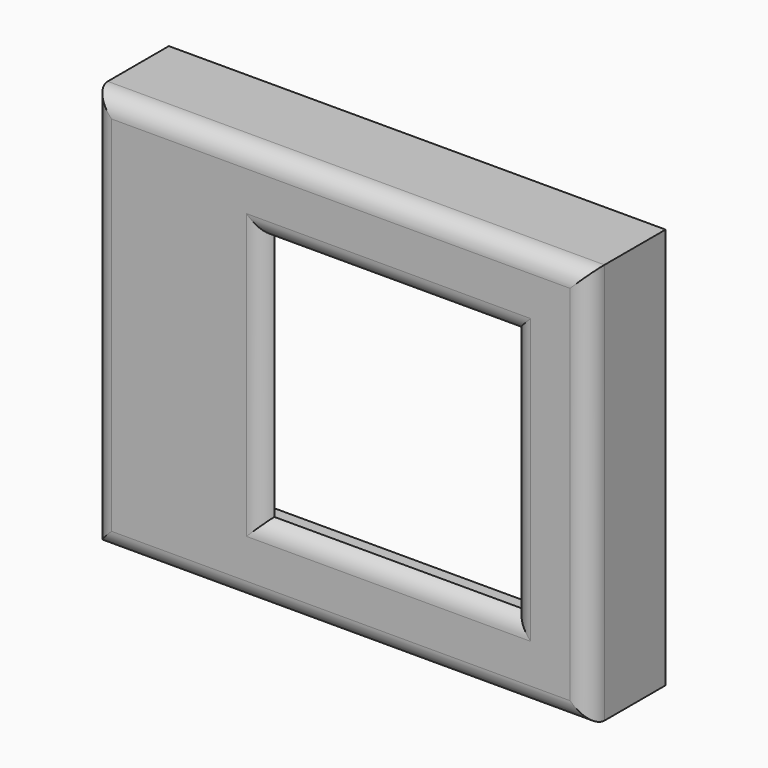
from build123d import *

# Parameters (mm, degrees)
F0_W         = 52
F0_H         = 42
F1_DEPTH     = 10
F2_W         = 26
F2_H         = 26
F3_DEPTH     = 25
F4_W         = 43
F4_H         = 36
F4_W_2       = 26
F4_H_2       = 26
F5_DEPTH     = 8.7
F6_T1_DEPTH  = 52
F6_T3_DEPTH  = 62
F6_T5_DEPTH  = 26
F6_T7_DEPTH  = 26
F6_T13_DEPTH = 30.6837484988
F6_T17_DEPTH = 30.6837484988
F6_T24_DEPTH = 30.6837484988
F6_T28_DEPTH = 30.6837484988
F6_T35_DEPTH = 30.6837484988
F6_T39_DEPTH = 30.6837484988
F6_T46_DEPTH = 30.6837484988
F6_T50_DEPTH = 30.6837484988


# Not quite as in the source:
# - a fillet or chamfer that OpenCascade refuses, or shapes differently, is made with other operations: its cross-section is extruded or revolved along the edge and cut away or added


with BuildPart() as f1:
    # F0 (on Front) → F1 (new body)
    with BuildSketch(Plane.XZ):
        Rectangle(F0_W, F0_H)
    extrude(amount=-F1_DEPTH)

    # F2 (on face) → F3 (cut)
    with BuildSketch(Plane.XZ):
        with Locations((5, 0)):
            Rectangle(F2_W, F2_H)
    extrude(amount=-F3_DEPTH, mode=Mode.SUBTRACT)

    # F4 (on face) → F5 (cut)
    with BuildSketch(Plane(origin=(0, 10, 0), x_dir=(-1, 0, 0), z_dir=(0, 1, 0))):
        with Locations((-1.5, 0)):
            Rectangle(F4_W, F4_H)
        with Locations((-5, 0)):
            Rectangle(F4_W_2, F4_H_2, mode=Mode.SUBTRACT)
    extrude(amount=-F5_DEPTH, mode=Mode.SUBTRACT)

    # F6: fillet of radius 2 on 8 edges, made by hand

    # F6_s2 → F6_t1 (cut)
    with BuildSketch(Plane.XY.offset(-26)):
        with BuildLine():
            ThreePointArc((-26, 2), (-25.4142135624, 0.5857864376), (-24, 0))
            Line((-24, 0), (-26, 0))
            Line((-26, 0), (-26, 2))
        make_face()
        with BuildLine():
            ThreePointArc((26, 2), (25.4142135624, 0.5857864376), (24, 0))
            Line((24, 0), (26, 0))
            Line((26, 0), (26, 2))
        make_face()
    extrude(amount=F6_T1_DEPTH, mode=Mode.SUBTRACT)

    # F6_s4 → F6_t3 (cut)
    with BuildSketch(Plane.YZ.offset(-31)):
        with BuildLine():
            ThreePointArc((0, 19), (0.5857864376, 20.4142135624), (2, 21))
            Line((2, 21), (0, 21))
            Line((0, 21), (0, 19))
        make_face()
        with BuildLine():
            ThreePointArc((2, -21), (0.5857864376, -20.4142135624), (0, -19))
            Line((0, -19), (0, -21))
            Line((0, -21), (2, -21))
        make_face()
    extrude(amount=F6_T3_DEPTH, mode=Mode.SUBTRACT)

    # F6_s6 → F6_t5 (cut)
    with BuildSketch(Plane.XY.offset(-13)):
        with BuildLine():
            ThreePointArc((-9.8734993995, 0), (-8.7333239744, 0.3568323275), (-8, 1.3))
            Line((-8, 1.3), (-8, 0))
            Line((-8, 0), (-9.8734993995, 0))
        make_face()
        with BuildLine():
            ThreePointArc((19.8734993995, 0), (18.7333239744, 0.3568323275), (18, 1.3))
            Line((18, 1.3), (18, 0))
            Line((18, 0), (19.8734993995, 0))
        make_face()
    extrude(amount=F6_T5_DEPTH, mode=Mode.SUBTRACT)

    # F6_s8 → F6_t7 (cut)
    with BuildSketch(Plane.YZ.offset(-8)):
        with BuildLine():
            ThreePointArc((0, -14.8734993995), (0.3568323275, -13.7333239744), (1.3, -13))
            Line((1.3, -13), (0, -13))
            Line((0, -13), (0, -14.8734993995))
        make_face()
        with BuildLine():
            ThreePointArc((0, 14.8734993995), (0.3568323275, 13.7333239744), (1.3, 13))
            Line((1.3, 13), (0, 13))
            Line((0, 13), (0, 14.8734993995))
        make_face()
    extrude(amount=F6_T7_DEPTH, mode=Mode.SUBTRACT)


with BuildPart() as f6_tool11:
    # F6_s12 → F6_t13 (new body)
    with BuildSketch(Plane.YZ.offset(18)):
        with BuildLine():
            ThreePointArc((0, 14.8734993995), (0.3568323275, 13.7333239744), (1.3, 13))
            Line((1.3, 13), (0, 13))
            Line((0, 13), (0, 14.8734993995))
        make_face()
    extrude(amount=-F6_T13_DEPTH)

    split(bisect_by=Plane.YZ.offset(-8), keep=Keep.BOTTOM)


with BuildPart() as f6_tool15:
    # F6_s16 → F6_t17 (new body)
    with BuildSketch(Plane.XY.offset(17.6837484988)):
        with BuildLine():
            ThreePointArc((-9.8734993995, 0), (-8.7333239744, 0.3568323275), (-8, 1.3))
            Line((-8, 1.3), (-8, 0))
            Line((-8, 0), (-9.8734993995, 0))
        make_face()
    extrude(amount=-F6_T17_DEPTH)

    split(bisect_by=Plane.XY.offset(13), keep=Keep.TOP)


with BuildPart() as f6_tool11_1:
    add(f6_tool11.part)

    # F6_t19: intersect F6_tool15
    add(f6_tool15.part, mode=Mode.INTERSECT)


with BuildPart() as f1_1:
    add(f1.part)

    # F6_t9: cut F6_tool11
    add(f6_tool11_1.part, mode=Mode.SUBTRACT)


with BuildPart() as f6_tool22:
    # F6_s23 → F6_t24 (new body)
    with BuildSketch(Plane.XY.offset(13)):
        with BuildLine():
            ThreePointArc((-9.8734993995, 0), (-8.7333239744, 0.3568323275), (-8, 1.3))
            Line((-8, 1.3), (-8, 0))
            Line((-8, 0), (-9.8734993995, 0))
        make_face()
    extrude(amount=-F6_T24_DEPTH)

    split(bisect_by=Plane.XY.offset(-13), keep=Keep.BOTTOM)


with BuildPart() as f6_tool26:
    # F6_s27 → F6_t28 (new body)
    with BuildSketch(Plane.YZ.offset(-12.6837484988)):
        with BuildLine():
            ThreePointArc((0, -14.8734993995), (0.3568323275, -13.7333239744), (1.3, -13))
            Line((1.3, -13), (0, -13))
            Line((0, -13), (0, -14.8734993995))
        make_face()
    extrude(amount=F6_T28_DEPTH)

    split(bisect_by=Plane.YZ.offset(-8), keep=Keep.BOTTOM)


with BuildPart() as f6_tool22_1:
    add(f6_tool22.part)

    # F6_t30: intersect F6_tool26
    add(f6_tool26.part, mode=Mode.INTERSECT)


with BuildPart() as f1_2:
    add(f1_1.part)

    # F6_t20: cut F6_tool22
    add(f6_tool22_1.part, mode=Mode.SUBTRACT)


with BuildPart() as f6_tool33:
    # F6_s34 → F6_t35 (new body)
    with BuildSketch(Plane.XY.offset(-17.6837484988)):
        with BuildLine():
            ThreePointArc((19.8734993995, 0), (18.7333239744, 0.3568323275), (18, 1.3))
            Line((18, 1.3), (18, 0))
            Line((18, 0), (19.8734993995, 0))
        make_face()
    extrude(amount=F6_T35_DEPTH)

    split(bisect_by=Plane.XY.offset(-13), keep=Keep.BOTTOM)


with BuildPart() as f6_tool37:
    # F6_s38 → F6_t39 (new body)
    with BuildSketch(Plane.YZ.offset(-8)):
        with BuildLine():
            ThreePointArc((0, -14.8734993995), (0.3568323275, -13.7333239744), (1.3, -13))
            Line((1.3, -13), (0, -13))
            Line((0, -13), (0, -14.8734993995))
        make_face()
    extrude(amount=F6_T39_DEPTH)

    split(bisect_by=Plane.YZ.offset(18), keep=Keep.TOP)


with BuildPart() as f6_tool33_1:
    add(f6_tool33.part)

    # F6_t41: intersect F6_tool37
    add(f6_tool37.part, mode=Mode.INTERSECT)


with BuildPart() as f1_3:
    add(f1_2.part)

    # F6_t31: cut F6_tool33
    add(f6_tool33_1.part, mode=Mode.SUBTRACT)


with BuildPart() as f6_tool44:
    # F6_s45 → F6_t46 (new body)
    with BuildSketch(Plane.XY.offset(-13)):
        with BuildLine():
            ThreePointArc((19.8734993995, 0), (18.7333239744, 0.3568323275), (18, 1.3))
            Line((18, 1.3), (18, 0))
            Line((18, 0), (19.8734993995, 0))
        make_face()
    extrude(amount=F6_T46_DEPTH)

    split(bisect_by=Plane.XY.offset(13), keep=Keep.TOP)


with BuildPart() as f6_tool48:
    # F6_s49 → F6_t50 (new body)
    with BuildSketch(Plane.YZ.offset(22.6837484988)):
        with BuildLine():
            ThreePointArc((0, 14.8734993995), (0.3568323275, 13.7333239744), (1.3, 13))
            Line((1.3, 13), (0, 13))
            Line((0, 13), (0, 14.8734993995))
        make_face()
    extrude(amount=-F6_T50_DEPTH)

    split(bisect_by=Plane.YZ.offset(18), keep=Keep.TOP)


with BuildPart() as f6_tool44_1:
    add(f6_tool44.part)

    # F6_t52: intersect F6_tool48
    add(f6_tool48.part, mode=Mode.INTERSECT)


with BuildPart() as f1_4:
    add(f1_3.part)

    # F6_t42: cut F6_tool44
    add(f6_tool44_1.part, mode=Mode.SUBTRACT)


solid = f1_4.part
